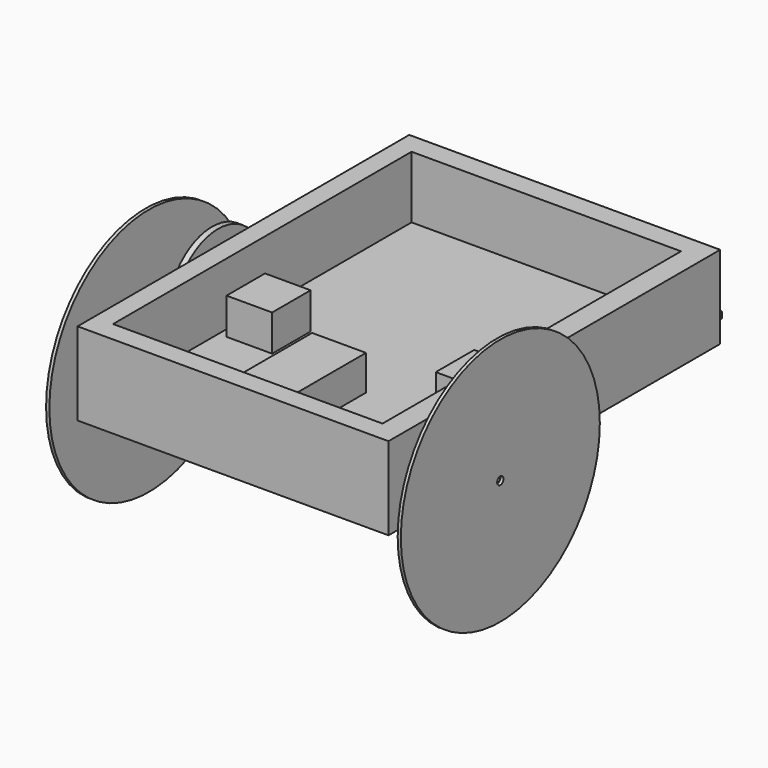
from build123d import *

# Parameters (mm, degrees)
F0_W      = 150
F0_H      = 200
F0_W_2    = 130
F0_H_2    = 180
F0_W_3    = 26
F0_H_3    = 44.7
F1_DEPTH  = 10
F3_START  = 75.65658
F2_R      = 60
F2_R_2    = 1.9010687787
F3_DEPTH  = 1.51959
F7_START  = 44.24528
F6_R      = 1.9348660317
F7_DEPTH  = 27.42483
F8_START  = -63.40283
F8_DEPTH  = 25.7397
F10_W     = 22
F10_H     = 23.2
F11_DEPTH = 27.5
F12_DEPTH = 40
F13_START = -92.37699
F13_DEPTH = 1.58359
F14_DEPTH = 26.9
F15_START = 66.3657
F9_R      = 27.2310204956
F15_DEPTH = 3.30842
F9_R_2    = 7.2888669106
F16_START = -84.74878
F16_DEPTH = 2.88128
F18_START = -113.94005
F17_W     = 38.7150868773
F17_H     = 2.9439013451
F18_DEPTH = 2.02893
F17_W_2   = 40.5191965401
F17_H_2   = 3.1723510474
F20_START = -100.74361
F19_W     = 3.284920007
F19_H     = 3.2849162817
F20_DEPTH = 14.37931
F19_W_2   = 2.5810077786
F19_H_2   = 3.0502793379


# Not quite as in the source:
# - the program builds the solid bodies; features that only make, move or delete a surface that nothing else refers to are left out


with BuildPart() as f1:
    # F0 (on Top) → F1 (new body)
    with BuildSketch(Plane.XY):
        with Locations((-9.2696487904, 6.2885135242)):
            Rectangle(F0_W, F0_H)
        with Locations((-10.0039294362, 6.098870337)):
            Rectangle(F0_W_2, F0_H_2, mode=Mode.SUBTRACT)
        with Locations((-10.0039294362, 6.098870337)):
            Rectangle(F0_W_2, F0_H_2)
        with Locations((-14.6333261281, -45.4308299661)):
            Rectangle(F0_W_3, F0_H_3, mode=Mode.SUBTRACT)
    extrude(amount=F1_DEPTH)

    # F10 (on Top) → F11 (join)
    with BuildSketch(Plane.XY):
        Polygon((-71.0902935837, -9.8448516801), (-71.0902935837, -20.3584678368), (-49.0902935837, -20.3584678368), (-49.0902935837, 2.8415321632), (-71.0902935837, 2.8415321632), (-71.0902935837, -7.195668295), align=None)
        with Locations((40.4238908535, -8.2341439949)):
            Rectangle(F10_W, F10_H)
    extrude(amount=F11_DEPTH)

    # F0 (on Top) → F12 (join)
    with BuildSketch(Plane.XY):
        with Locations((-9.2696487904, 6.2885135242)):
            Rectangle(F0_W, F0_H)
        with Locations((-10.0039294362, 6.098870337)):
            Rectangle(F0_W_2, F0_H_2, mode=Mode.SUBTRACT)
    extrude(amount=F12_DEPTH)

    # F0 (on Top) → F14 (join)
    with BuildSketch(Plane.XY):
        with Locations((-14.6333261281, -45.4308299661)):
            Rectangle(F0_W_3, F0_H_3)
    extrude(amount=F14_DEPTH)


with BuildPart() as f3:
    # F2 (on Right) → F3 (new body)
    with BuildSketch(Plane.YZ.offset(F3_START)):
        with Locations((-40.5887551606, 5.3735026158)):
            Circle(F2_R)
        with Locations((-40.5887551606, 5.3735026158)):
            Circle(F2_R_2, mode=Mode.SUBTRACT)
    extrude(amount=F3_DEPTH)


with BuildPart() as f7:
    # F6 (on Right) → F7 (new body)
    with BuildSketch(Plane.YZ.offset(F7_START)):
        with Locations((-8.6473254487, 19.3343963474)):
            Circle(F6_R)
    extrude(amount=F7_DEPTH)

    # F9 (on Right) → F15 (join)
    with BuildSketch(Plane.YZ.offset(F15_START)):
        with Locations((-8.4126899019, 19.3343963474)):
            Circle(F9_R)
    extrude(amount=F15_DEPTH)


with BuildPart() as f8:
    # F6 (on Right) → F8 (new body)
    with BuildSketch(Plane.YZ.offset(F8_START)):
        with Locations((-8.6473254487, 19.3343963474)):
            Circle(F6_R)
    extrude(amount=-F8_DEPTH)

    # F9 (on Right) → F16 (join)
    with BuildSketch(Plane.YZ.offset(F16_START)):
        with Locations((-8.4126899019, 19.3343963474)):
            Circle(F9_R)
    extrude(amount=-F16_DEPTH)


with BuildPart() as f13:
    # F2 (on Right) → F13 (new body)
    with BuildSketch(Plane.YZ.offset(F13_START)):
        with Locations((-40.5887551606, 5.3735026158)):
            Circle(F2_R)
        with Locations((-40.5887551606, 5.3735026158)):
            Circle(F2_R_2, mode=Mode.SUBTRACT)
    extrude(amount=-F13_DEPTH)


with BuildPart() as f15:
    # F9 (on Right) → F15, piece 2 (new body)
    with BuildSketch(Plane.YZ.offset(F15_START)):
        with Locations((-40.5579395592, 5.4908203892)):
            Circle(F9_R_2)
    extrude(amount=F15_DEPTH)


with BuildPart() as f16:
    # F9 (on Right) → F16, piece 2 (new body)
    with BuildSketch(Plane.YZ.offset(F16_START)):
        with Locations((-40.5579395592, 5.4908203892)):
            Circle(F9_R_2)
    extrude(amount=-F16_DEPTH)


with BuildPart() as f18:
    # F17 (on Front) → F18 (new body)
    with BuildSketch(Plane.XZ.offset(F18_START)):
        with Locations((39.4729152322, 6.1306017451)):
            Rectangle(F17_W, F17_H)
    extrude(amount=-F18_DEPTH)


with BuildPart() as f18b:
    # F17 (on Front) → F18, piece 2 (new body)
    with BuildSketch(Plane.XZ.offset(F18_START)):
        with Locations((-54.4183310121, 6.2448265962)):
            Rectangle(F17_W_2, F17_H_2)
    extrude(amount=-F18_DEPTH)


with BuildPart() as f20:
    # F19 (on Front) → F20 (new body)
    with BuildSketch(Plane.XZ.offset(F20_START)):
        with Locations((57.1879986674, 5.9600942768)):
            Rectangle(F19_W, F19_H)
    extrude(amount=-F20_DEPTH)


with BuildPart() as f20b:
    # F19 (on Front) → F20, piece 2 (new body)
    with BuildSketch(Plane.XZ.offset(F20_START)):
        with Locations((-73.1527842581, 6.0774127487)):
            Rectangle(F19_W_2, F19_H_2)
    extrude(amount=-F20_DEPTH)


solid = Compound([f1.part, f3.part, f7.part, f8.part, f13.part, f15.part, f16.part, f18.part, f18b.part, f20.part, f20b.part])
